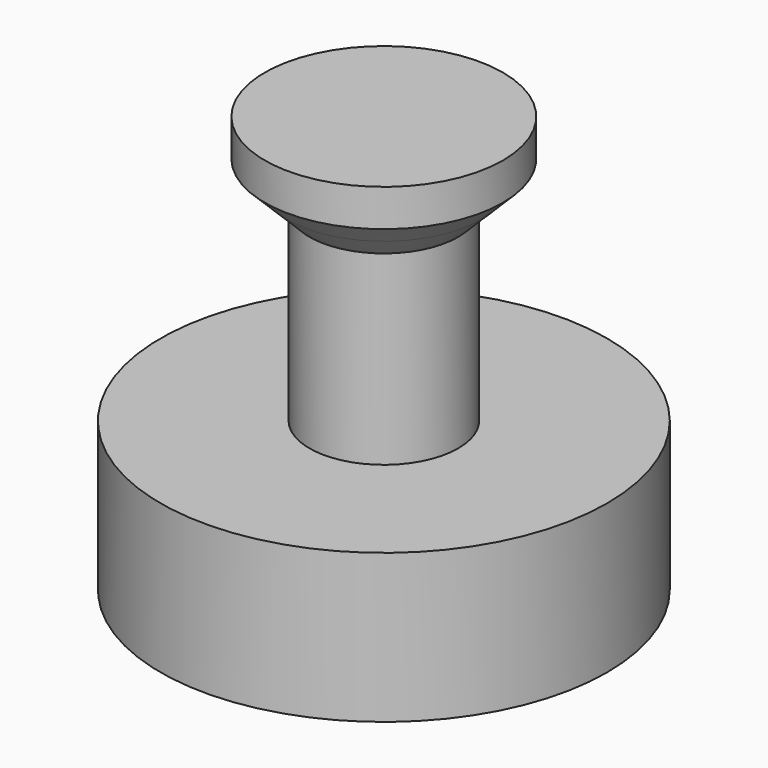
from build123d import *

# Parameters (mm, degrees)
F6_R      = 2.5
F7_DEPTH  = 12
F6_R_2    = 7.5
F8_DEPTH  = 5
F9_R      = 4
F9_R_2    = 2.5
F10_DEPTH = 2
F11_SIZE  = 0.74999


# Not quite as in the source:
# - a fillet or chamfer is up to 0.001 mm smaller than in the source, because OpenCascade refuses the exact size


with BuildPart() as f7:
    # F6 (on Top) → F7 (new body)
    with BuildSketch(Plane.XY):
        Circle(F6_R)
    extrude(amount=F7_DEPTH)

    # F6 (on Top) → F8 (join)
    with BuildSketch(Plane.XY):
        Circle(F6_R_2)
        Circle(F6_R, mode=Mode.SUBTRACT)
    extrude(amount=F8_DEPTH)

    # F9 (on face) → F10 (join)
    with BuildSketch(Plane.XY.offset(12)):
        Circle(F9_R)
        Circle(F9_R_2, mode=Mode.SUBTRACT)
        Circle(F9_R_2)
    extrude(amount=F10_DEPTH)

    # F11 (size 0.75 in the source; OpenCascade refuses exactly that, so slightly less here)
    f11_edges = [f7.edges().sort_by_distance(p)[0] for p in [
        (-4, 0, 12),
        (-2.5, 0, 12),
    ]]
    chamfer(f11_edges, length=F11_SIZE)


solid = f7.part
